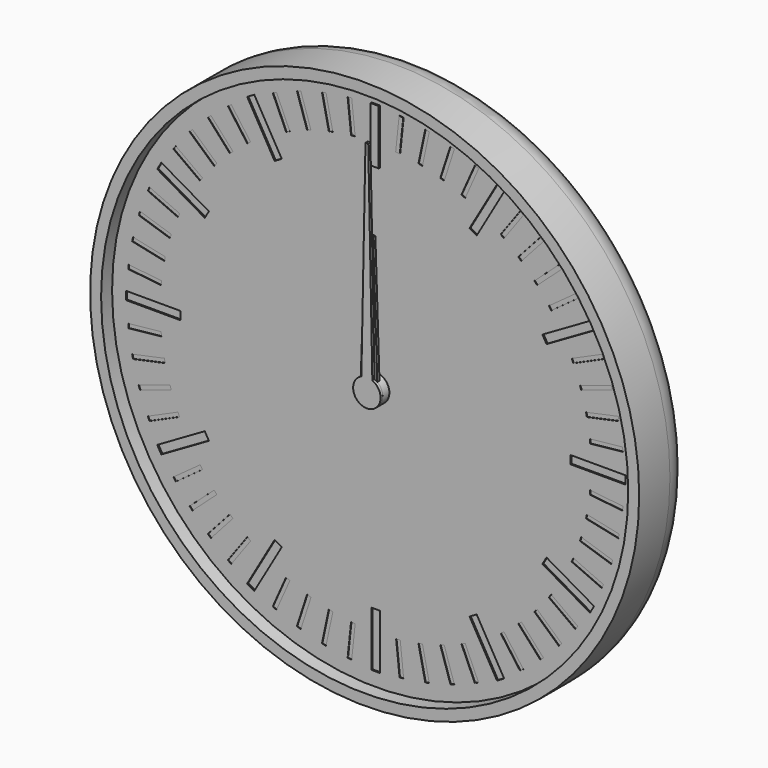
from build123d import *

# Parameters (mm, degrees)
F0_R      = 100
F1_DEPTH  = 24
F2_R      = 10
F3_T      = -4
F4_R      = 5
F4_R_2    = 3
F5_DEPTH  = 2
F6_DEPTH  = 19
F7_DEPTH  = 8
F9_DEPTH  = 4
F11_DEPTH = 4
F12_R     = 5
F12_R_2   = 3
F13_DEPTH = 2
F14_R     = 3
F15_DEPTH = 4
F17_DEPTH = 4
F18_R     = 3
F19_DEPTH = 2
F20_R     = 98
F20_R_2   = 5
F21_DEPTH = 1
F23_R     = 5
F23_R_2   = 3
F24_DEPTH = 2
F25_W     = 3
F25_H     = 20
F25_W_2   = 20
F25_H_2   = 3
F26_DEPTH = 0.5
F27_W     = 1.5
F27_H     = 12
F27_W_2   = 12
F27_H_2   = 1.5
F28_DEPTH = 0.2
F29_DEPTH = 1
F30_DEPTH = 0.4
F31_R     = 5
F31_R_2   = 3
F32_DEPTH = 5
F33_R     = 3
F34_DEPTH = 1
F36_DEPTH = 1


with BuildPart() as f1:
    # F0 (on Front) → F1 (new body)
    with BuildSketch(Plane.XZ):
        Circle(F0_R)
    extrude(amount=F1_DEPTH)

    # F2
    f2_edges = [f1.edges().sort_by_distance(p)[0] for p in [
        (-100, 0, 0),
    ]]
    fillet(f2_edges, radius=F2_R)

    # F3
    f3_openings = [f1.faces().sort_by_distance(p)[0] for p in [
        (0, -24, 0),
    ]]
    offset(amount=F3_T, openings=f3_openings)

    # F4 (on face) → F5 (join)
    with BuildSketch(Plane.XZ.offset(4)):
        Circle(F4_R)
        Circle(F4_R_2, mode=Mode.SUBTRACT)
        with Locations((40, 0)):
            Circle(F4_R)
        with Locations((40, 0)):
            Circle(F4_R_2, mode=Mode.SUBTRACT)
    extrude(amount=F5_DEPTH)


with BuildPart() as f6:
    # F6 (new): a face of the model
    f6_faces = [f1.part.faces().sort_by_distance(p)[0] for p in [
        (0, -4, 0),
    ]]
    extrude(f6_faces, amount=F6_DEPTH)

    # F8 (on face) → F9 (join)
    with BuildSketch(Plane.XZ.offset(6)):
        with BuildLine():
            ThreePointArc((9.2729637667, -1.3794085621), (9.3494561423, -0.6915886375), (9.375, 0))
            ThreePointArc((9.375, 0), (9.3494561423, 0.6915886375), (9.2729637667, 1.3794085621))
            ThreePointArc((9.2729637667, 1.3794085621), (8.9161548403, 2.8970343223), (8.3127812852, 4.3345463782))
            ThreePointArc((8.3127812852, 4.3345463782), (7.5845343223, 5.5104867402), (6.6911892658, 6.566476316))
            ThreePointArc((6.6911892658, 6.566476316), (5.5104867402, 7.5845343223), (4.1773988938, 8.3928519278))
            ThreePointArc((4.1773988938, 8.3928519278), (2.8970343223, 8.9161548403), (1.5536078905, 9.2453733036))
            ThreePointArc((1.5536078905, 9.2453733036), (0, 9.375), (-1.5536078905, 9.2453733036))
            ThreePointArc((-1.5536078905, 9.2453733036), (-2.8970343223, 8.9161548403), (-4.1773988938, 8.3928519278))
            ThreePointArc((-4.1773988938, 8.3928519278), (-5.5104867402, 7.5845343223), (-6.6911892658, 6.566476316))
            ThreePointArc((-6.6911892658, 6.566476316), (-7.5845343223, 5.5104867402), (-8.3127812852, 4.3345463782))
            ThreePointArc((-8.3127812852, 4.3345463782), (-8.9161548403, 2.8970343223), (-9.2729637667, 1.3794085621))
            ThreePointArc((-9.2729637667, 1.3794085621), (-9.375, 0), (-9.2729637667, -1.3794085621))
            ThreePointArc((-9.2729637667, -1.3794085621), (-8.9161548403, -2.8970343223), (-8.3127812852, -4.3345463782))
            ThreePointArc((-8.3127812852, -4.3345463782), (-7.5845343223, -5.5104867402), (-6.6911892658, -6.566476316))
            ThreePointArc((-6.6911892658, -6.566476316), (-5.5104867402, -7.5845343223), (-4.1773988938, -8.3928519278))
            ThreePointArc((-4.1773988938, -8.3928519278), (-2.8970343223, -8.9161548403), (-1.5536078905, -9.2453733036))
            ThreePointArc((-1.5536078905, -9.2453733036), (0, -9.375), (1.5536078905, -9.2453733036))
            ThreePointArc((1.5536078905, -9.2453733036), (2.8970343223, -8.9161548403), (4.1773988938, -8.3928519278))
            ThreePointArc((4.1773988938, -8.3928519278), (5.5104867402, -7.5845343223), (6.6911892658, -6.566476316))
            ThreePointArc((6.6911892658, -6.566476316), (7.5845343223, -5.5104867402), (8.3127812852, -4.3345463782))
            ThreePointArc((8.3127812852, -4.3345463782), (8.9161548403, -2.8970343223), (9.2729637667, -1.3794085621))
        make_face()
        with BuildLine():
            ThreePointArc((8.3127812852, 4.3345463782), (8.9161548403, 2.8970343223), (9.2729637667, 1.3794085621))
            Line((9.2729637667, 1.3794085621), (11.1823199426, 2.3946312492))
            Line((11.1823199426, 2.3946312492), (10.8182678729, 3.515068311))
            Line((10.8182678729, 3.515068311), (10.4542158031, 4.6355053728))
            Line((10.4542158031, 4.6355053728), (8.3127812852, 4.3345463782))
        make_face()
        with BuildLine():
            Line((11.1823199426, -2.3946312492), (9.2729637667, -1.3794085621))
            ThreePointArc((9.2729637667, -1.3794085621), (8.9161548403, -2.8970343223), (8.3127812852, -4.3345463782))
            Line((8.3127812852, -4.3345463782), (10.4542158031, -4.6355053728))
            Line((10.4542158031, -4.6355053728), (10.8182678729, -3.515068311))
            Line((10.8182678729, -3.515068311), (11.1823199426, -2.3946312492))
        make_face()
        with BuildLine():
            ThreePointArc((4.1773988938, 8.3928519278), (5.5104867402, 7.5845343223), (6.6911892658, 6.566476316))
            Line((6.6911892658, 6.566476316), (7.6391579371, 8.5101001246))
            Line((7.6391579371, 8.5101001246), (6.6860572448, 9.202568311))
            Line((6.6860572448, 9.202568311), (5.7329565525, 9.8950364974))
            Line((5.7329565525, 9.8950364974), (4.1773988938, 8.3928519278))
        make_face()
        with BuildLine():
            Line((7.6391579371, -8.5101001246), (6.6911892658, -6.566476316))
            ThreePointArc((6.6911892658, -6.566476316), (5.5104867402, -7.5845343223), (4.1773988938, -8.3928519278))
            Line((4.1773988938, -8.3928519278), (5.7329565525, -9.8950364974))
            Line((5.7329565525, -9.8950364974), (6.6860572448, -9.202568311))
            Line((6.6860572448, -9.202568311), (7.6391579371, -8.5101001246))
        make_face()
        with BuildLine():
            ThreePointArc((-1.5536078905, 9.2453733036), (0, 9.375), (1.5536078905, 9.2453733036))
            Line((1.5536078905, 9.2453733036), (1.1780972451, 11.375))
            Line((1.1780972451, 11.375), (0, 11.375))
            Line((0, 11.375), (-1.1780972451, 11.375))
            Line((-1.1780972451, 11.375), (-1.5536078905, 9.2453733036))
        make_face()
        with BuildLine():
            Line((1.1780972451, -11.375), (1.5536078905, -9.2453733036))
            ThreePointArc((1.5536078905, -9.2453733036), (0, -9.375), (-1.5536078905, -9.2453733036))
            Line((-1.5536078905, -9.2453733036), (-1.1780972451, -11.375))
            Line((-1.1780972451, -11.375), (0, -11.375))
            Line((0, -11.375), (1.1780972451, -11.375))
        make_face()
        with BuildLine():
            ThreePointArc((-6.6911892658, 6.566476316), (-5.5104867402, 7.5845343223), (-4.1773988938, 8.3928519278))
            Line((-4.1773988938, 8.3928519278), (-5.7329565525, 9.8950364974))
            Line((-5.7329565525, 9.8950364974), (-6.6860572448, 9.202568311))
            Line((-6.6860572448, 9.202568311), (-7.6391579371, 8.5101001246))
            Line((-7.6391579371, 8.5101001246), (-6.6911892658, 6.566476316))
        make_face()
        with BuildLine():
            Line((-5.7329565525, -9.8950364974), (-4.1773988938, -8.3928519278))
            ThreePointArc((-4.1773988938, -8.3928519278), (-5.5104867402, -7.5845343223), (-6.6911892658, -6.566476316))
            Line((-6.6911892658, -6.566476316), (-7.6391579371, -8.5101001246))
            Line((-7.6391579371, -8.5101001246), (-6.6860572448, -9.202568311))
            Line((-6.6860572448, -9.202568311), (-5.7329565525, -9.8950364974))
        make_face()
        with BuildLine():
            ThreePointArc((-9.2729637667, 1.3794085621), (-8.9161548403, 2.8970343223), (-8.3127812852, 4.3345463782))
            Line((-8.3127812852, 4.3345463782), (-10.4542158031, 4.6355053728))
            Line((-10.4542158031, 4.6355053728), (-10.8182678729, 3.515068311))
            Line((-10.8182678729, 3.515068311), (-11.1823199426, 2.3946312492))
            Line((-11.1823199426, 2.3946312492), (-9.2729637667, 1.3794085621))
        make_face()
        with BuildLine():
            Line((-10.4542158031, -4.6355053728), (-8.3127812852, -4.3345463782))
            ThreePointArc((-8.3127812852, -4.3345463782), (-8.9161548403, -2.8970343223), (-9.2729637667, -1.3794085621))
            Line((-9.2729637667, -1.3794085621), (-11.1823199426, -2.3946312492))
            Line((-11.1823199426, -2.3946312492), (-10.8182678729, -3.515068311))
            Line((-10.8182678729, -3.515068311), (-10.4542158031, -4.6355053728))
        make_face()
    extrude(amount=F9_DEPTH)

    # F35 (on face) → F36 (join)
    with BuildSketch(Plane.XZ.offset(23)):
        with BuildLine():
            ThreePointArc((-2, 4.582575695), (-2.7386127875, -4.1833001327), (5, 0))
            ThreePointArc((5, 0), (4.1833001327, 2.7386127875), (2, 4.582575695))
            ThreePointArc((2, 4.582575695), (0, 5), (-2, 4.582575695))
        make_face()
        with BuildLine():
            ThreePointArc((-2, 4.582575695), (0, 5), (2, 4.582575695))
            Line((2, 4.582575695), (0.5, 80))
            Line((0.5, 80), (0, 80))
            Line((0, 80), (-0.5, 80))
            Line((-0.5, 80), (-2, 4.582575695))
        make_face()
    extrude(amount=-F36_DEPTH)


with BuildPart() as f7:
    # F7 (new): a face of the model
    f7_faces = [f1.part.faces().sort_by_distance(p)[0] for p in [
        (40, -4, 0),
    ]]
    extrude(f7_faces, amount=F7_DEPTH)

    # F10 (on face) → F11 (join)
    with BuildSketch(Plane.XZ.offset(6)):
        with BuildLine():
            ThreePointArc((68.0829066802, -1.5381733945), (68.1144747006, -0.7693746225), (68.125, 0))
            ThreePointArc((68.125, 0), (68.1144747006, 0.7693746225), (68.0829066802, 1.5381733945))
            ThreePointArc((68.0829066802, 1.5381733945), (67.9709283072, 2.9398630294), (67.7890320221, 4.3342039956))
            ThreePointArc((67.7890320221, 4.3342039956), (67.5104012706, 5.8475163042), (67.1494235596, 7.3433252263))
            ThreePointArc((67.1494235596, 7.3433252263), (66.7484645208, 8.6911029668), (66.280643318, 10.0171558733))
            ThreePointArc((66.280643318, 10.0171558733), (65.6934659962, 11.4394680865), (65.0293803521, 12.8275385085))
            ThreePointArc((65.0293803521, 12.8275385085), (64.3569644814, 14.0625), (63.6236643925, 15.2623099717))
            ThreePointArc((63.6236643925, 15.2623099717), (62.7536029668, 16.5314602207), (61.815433119, 17.7511268046))
            ThreePointArc((61.815433119, 17.7511268046), (60.9009482166, 18.8192983038), (59.934217974, 19.8404278876))
            ThreePointArc((59.934217974, 19.8404278876), (58.8192983038, 20.9009482166), (57.6480467764, 21.8989056799))
            ThreePointArc((57.6480467764, 21.8989056799), (56.5314602207, 22.7536029668), (55.3735505752, 23.5514238999))
            ThreePointArc((55.3735505752, 23.5514238999), (54.0625, 24.3569644814), (52.709356105, 25.0895972944))
            ThreePointArc((52.709356105, 25.0895972944), (51.4394680865, 25.6934659962), (50.1409852457, 26.2331096755))
            ThreePointArc((50.1409852457, 26.2331096755), (48.6911029668, 26.7484645208), (47.2152055856, 27.1837531139))
            ThreePointArc((47.2152055856, 27.1837531139), (45.8475163042, 27.5104012706), (44.4652101991, 27.7682826779))
            ThreePointArc((44.4652101991, 27.7682826779), (42.9398630294, 27.9709283072), (41.4057159597, 28.0898484802))
            ThreePointArc((41.4057159597, 28.0898484802), (40, 28.125), (38.5942840403, 28.0898484802))
            ThreePointArc((38.5942840403, 28.0898484802), (37.0601369706, 27.9709283072), (35.5347898009, 27.7682826779))
            ThreePointArc((35.5347898009, 27.7682826779), (34.1524836958, 27.5104012706), (32.7847944144, 27.1837531139))
            ThreePointArc((32.7847944144, 27.1837531139), (31.3088970332, 26.7484645208), (29.8590147543, 26.2331096755))
            ThreePointArc((29.8590147543, 26.2331096755), (28.5605319135, 25.6934659962), (27.290643895, 25.0895972944))
            ThreePointArc((27.290643895, 25.0895972944), (25.9375, 24.3569644814), (24.6264494248, 23.5514238999))
            ThreePointArc((24.6264494248, 23.5514238999), (23.4685397793, 22.7536029668), (22.3519532236, 21.8989056799))
            ThreePointArc((22.3519532236, 21.8989056799), (21.1807016962, 20.9009482166), (20.065782026, 19.8404278876))
            ThreePointArc((20.065782026, 19.8404278876), (19.0990517834, 18.8192983038), (18.184566881, 17.7511268046))
            ThreePointArc((18.184566881, 17.7511268046), (17.2463970332, 16.5314602207), (16.3763356075, 15.2623099717))
            ThreePointArc((16.3763356075, 15.2623099717), (15.6430355186, 14.0625), (14.9706196479, 12.8275385085))
            ThreePointArc((14.9706196479, 12.8275385085), (14.3065340038, 11.4394680865), (13.719356682, 10.0171558733))
            ThreePointArc((13.719356682, 10.0171558733), (13.2515354792, 8.6911029668), (12.8505764404, 7.3433252263))
            ThreePointArc((12.8505764404, 7.3433252263), (12.4895987294, 5.8475163042), (12.2109679779, 4.3342039956))
            ThreePointArc((12.2109679779, 4.3342039956), (12.0290716928, 2.9398630294), (11.9170933198, 1.5381733945))
            ThreePointArc((11.9170933198, 1.5381733945), (11.875, 0), (11.9170933198, -1.5381733945))
            ThreePointArc((11.9170933198, -1.5381733945), (12.0290716928, -2.9398630294), (12.2109679779, -4.3342039956))
            ThreePointArc((12.2109679779, -4.3342039956), (12.4895987294, -5.8475163042), (12.8505764404, -7.3433252263))
            ThreePointArc((12.8505764404, -7.3433252263), (13.2515354792, -8.6911029668), (13.719356682, -10.0171558733))
            ThreePointArc((13.719356682, -10.0171558733), (14.3065340038, -11.4394680865), (14.9706196479, -12.8275385085))
            ThreePointArc((14.9706196479, -12.8275385085), (15.6430355186, -14.0625), (16.3763356075, -15.2623099717))
            ThreePointArc((16.3763356075, -15.2623099717), (17.2463970332, -16.5314602207), (18.184566881, -17.7511268046))
            ThreePointArc((18.184566881, -17.7511268046), (19.0990517834, -18.8192983038), (20.065782026, -19.8404278876))
            ThreePointArc((20.065782026, -19.8404278876), (21.1807016962, -20.9009482166), (22.3519532236, -21.8989056799))
            ThreePointArc((22.3519532236, -21.8989056799), (23.4685397793, -22.7536029668), (24.6264494248, -23.5514238999))
            ThreePointArc((24.6264494248, -23.5514238999), (25.9375, -24.3569644814), (27.290643895, -25.0895972944))
            ThreePointArc((27.290643895, -25.0895972944), (28.5605319135, -25.6934659962), (29.8590147543, -26.2331096755))
            ThreePointArc((29.8590147543, -26.2331096755), (31.3088970332, -26.7484645208), (32.7847944144, -27.1837531139))
            ThreePointArc((32.7847944144, -27.1837531139), (34.1524836958, -27.5104012706), (35.5347898009, -27.7682826779))
            ThreePointArc((35.5347898009, -27.7682826779), (37.0601369706, -27.9709283072), (38.5942840403, -28.0898484802))
            ThreePointArc((38.5942840403, -28.0898484802), (40, -28.125), (41.4057159597, -28.0898484802))
            ThreePointArc((41.4057159597, -28.0898484802), (42.9398630294, -27.9709283072), (44.4652101991, -27.7682826779))
            ThreePointArc((44.4652101991, -27.7682826779), (45.8475163042, -27.5104012706), (47.2152055856, -27.1837531139))
            ThreePointArc((47.2152055856, -27.1837531139), (48.6911029668, -26.7484645208), (50.1409852457, -26.2331096755))
            ThreePointArc((50.1409852457, -26.2331096755), (51.4394680865, -25.6934659962), (52.709356105, -25.0895972944))
            ThreePointArc((52.709356105, -25.0895972944), (54.0625, -24.3569644814), (55.3735505752, -23.5514238999))
            ThreePointArc((55.3735505752, -23.5514238999), (56.5314602207, -22.7536029668), (57.6480467764, -21.8989056799))
            ThreePointArc((57.6480467764, -21.8989056799), (58.8192983038, -20.9009482166), (59.934217974, -19.8404278876))
            ThreePointArc((59.934217974, -19.8404278876), (60.9009482166, -18.8192983038), (61.815433119, -17.7511268046))
            ThreePointArc((61.815433119, -17.7511268046), (62.7536029668, -16.5314602207), (63.6236643925, -15.2623099717))
            ThreePointArc((63.6236643925, -15.2623099717), (64.3569644814, -14.0625), (65.0293803521, -12.8275385085))
            ThreePointArc((65.0293803521, -12.8275385085), (65.6934659962, -11.4394680865), (66.280643318, -10.0171558733))
            ThreePointArc((66.280643318, -10.0171558733), (66.7484645208, -8.6911029668), (67.1494235596, -7.3433252263))
            ThreePointArc((67.1494235596, -7.3433252263), (67.5104012706, -5.8475163042), (67.7890320221, -4.3342039956))
            ThreePointArc((67.7890320221, -4.3342039956), (67.9709283072, -2.9398630294), (68.0829066802, -1.5381733945))
        make_face()
        with BuildLine():
            ThreePointArc((68.0829066802, 1.5381733945), (68.1144747006, 0.7693746225), (68.125, 0))
            ThreePointArc((68.125, 0), (68.1144747006, -0.7693746225), (68.0829066802, -1.5381733945))
            Line((68.0829066802, -1.5381733945), (70.125, -1.1780972451))
            Line((70.125, -1.1780972451), (70.125, 0))
            Line((70.125, 0), (70.125, 1.1780972451))
            Line((70.125, 1.1780972451), (68.0829066802, 1.5381733945))
        make_face()
        with BuildLine():
            ThreePointArc((67.1494235596, 7.3433252263), (67.5104012706, 5.8475163042), (67.7890320221, 4.3342039956))
            Line((67.7890320221, 4.3342039956), (69.7116366623, 5.1109866922))
            Line((69.7116366623, 5.1109866922), (69.4666964721, 6.2633396859))
            Line((69.4666964721, 6.2633396859), (69.2217562819, 7.4156926796))
            Line((69.2217562819, 7.4156926796), (67.1494235596, 7.3433252263))
        make_face()
        with BuildLine():
            Line((69.7116366623, -5.1109866922), (67.7890320221, -4.3342039956))
            ThreePointArc((67.7890320221, -4.3342039956), (67.5104012706, -5.8475163042), (67.1494235596, -7.3433252263))
            Line((67.1494235596, -7.3433252263), (69.2217562819, -7.4156926796))
            Line((69.2217562819, -7.4156926796), (69.4666964721, -6.2633396859))
            Line((69.4666964721, -6.2633396859), (69.7116366623, -5.1109866922))
        make_face()
        with BuildLine():
            ThreePointArc((65.0293803521, 12.8275385085), (65.6934659962, 11.4394680865), (66.280643318, 10.0171558733))
            Line((66.280643318, 10.0171558733), (67.9997322302, 11.1766959857))
            Line((67.9997322302, 11.1766959857), (67.5205569115, 12.2529413727))
            Line((67.5205569115, 12.2529413727), (67.0413815928, 13.3291867596))
            Line((67.0413815928, 13.3291867596), (65.0293803521, 12.8275385085))
        make_face()
        with BuildLine():
            Line((67.9997322302, -11.1766959857), (66.280643318, -10.0171558733))
            ThreePointArc((66.280643318, -10.0171558733), (65.6934659962, -11.4394680865), (65.0293803521, -12.8275385085))
            Line((65.0293803521, -12.8275385085), (67.0413815928, -13.3291867596))
            Line((67.0413815928, -13.3291867596), (67.5205569115, -12.2529413727))
            Line((67.5205569115, -12.2529413727), (67.9997322302, -11.1766959857))
        make_face()
        with BuildLine():
            ThreePointArc((61.815433119, 17.7511268046), (62.7536029668, 16.5314602207), (63.6236643925, 15.2623099717))
            Line((63.6236643925, 15.2623099717), (65.064105142, 16.753930033))
            Line((65.064105142, 16.753930033), (64.3716369555, 17.7070307253))
            Line((64.3716369555, 17.7070307253), (63.6791687691, 18.6601314176))
            Line((63.6791687691, 18.6601314176), (61.815433119, 17.7511268046))
        make_face()
        with BuildLine():
            Line((65.064105142, -16.753930033), (63.6236643925, -15.2623099717))
            ThreePointArc((63.6236643925, -15.2623099717), (62.7536029668, -16.5314602207), (61.815433119, -17.7511268046))
            Line((61.815433119, -17.7511268046), (63.6791687691, -18.6601314176))
            Line((63.6791687691, -18.6601314176), (64.3716369555, -17.7070307253))
            Line((64.3716369555, -17.7070307253), (65.064105142, -16.753930033))
        make_face()
        with BuildLine():
            ThreePointArc((57.6480467764, 21.8989056799), (58.8192983038, 20.9009482166), (59.934217974, 19.8404278876))
            Line((59.934217974, 19.8404278876), (61.0330563882, 21.5989369435))
            Line((61.0330563882, 21.5989369435), (60.1575595166, 22.3872378675))
            Line((60.1575595166, 22.3872378675), (59.282062645, 23.1755387915))
            Line((59.282062645, 23.1755387915), (57.6480467764, 21.8989056799))
        make_face()
        with BuildLine():
            Line((61.0330563882, -21.5989369435), (59.934217974, -19.8404278876))
            ThreePointArc((59.934217974, -19.8404278876), (58.8192983038, -20.9009482166), (57.6480467764, -21.8989056799))
            Line((57.6480467764, -21.8989056799), (59.282062645, -23.1755387915))
            Line((59.282062645, -23.1755387915), (60.1575595166, -22.3872378675))
            Line((60.1575595166, -22.3872378675), (61.0330563882, -21.5989369435))
        make_face()
        with BuildLine():
            ThreePointArc((52.709356105, 25.0895972944), (54.0625, 24.3569644814), (55.3735505752, 23.5514238999))
            Line((55.3735505752, 23.5514238999), (56.0827621424, 25.4999666665))
            Line((56.0827621424, 25.4999666665), (55.0625, 26.089015289))
            Line((55.0625, 26.089015289), (54.0422378576, 26.6780639116))
            Line((54.0422378576, 26.6780639116), (52.709356105, 25.0895972944))
        make_face()
        with BuildLine():
            Line((56.0827621424, -25.4999666665), (55.3735505752, -23.5514238999))
            ThreePointArc((55.3735505752, -23.5514238999), (54.0625, -24.3569644814), (52.709356105, -25.0895972944))
            Line((52.709356105, -25.0895972944), (54.0422378576, -26.6780639116))
            Line((54.0422378576, -26.6780639116), (55.0625, -26.089015289))
            Line((55.0625, -26.089015289), (56.0827621424, -25.4999666665))
        make_face()
        with BuildLine():
            ThreePointArc((47.2152055856, 27.1837531139), (48.6911029668, 26.7484645208), (50.1409852457, 26.2331096755))
            Line((50.1409852457, 26.2331096755), (50.4295740173, 28.2865254836))
            Line((50.4295740173, 28.2865254836), (49.3091369555, 28.6505775534))
            Line((49.3091369555, 28.6505775534), (48.1886998938, 29.0146296232))
            Line((48.1886998938, 29.0146296232), (47.2152055856, 27.1837531139))
        make_face()
        with BuildLine():
            Line((50.4295740173, -28.2865254836), (50.1409852457, -26.2331096755))
            ThreePointArc((50.1409852457, -26.2331096755), (48.6911029668, -26.7484645208), (47.2152055856, -27.1837531139))
            Line((47.2152055856, -27.1837531139), (48.1886998938, -29.0146296232))
            Line((48.1886998938, -29.0146296232), (49.3091369555, -28.6505775534))
            Line((49.3091369555, -28.6505775534), (50.4295740173, -28.2865254836))
        make_face()
        with BuildLine():
            ThreePointArc((41.4057159597, 28.0898484802), (42.9398630294, 27.9709283072), (44.4652101991, 27.7682826779))
            Line((44.4652101991, 27.7682826779), (44.3205634611, 29.8368274034))
            Line((44.3205634611, 29.8368274034), (43.1489199559, 29.959972098))
            Line((43.1489199559, 29.959972098), (41.9772764508, 30.0831167926))
            Line((41.9772764508, 30.0831167926), (41.4057159597, 28.0898484802))
        make_face()
        with BuildLine():
            Line((44.3205634611, -29.8368274034), (44.4652101991, -27.7682826779))
            ThreePointArc((44.4652101991, -27.7682826779), (42.9398630294, -27.9709283072), (41.4057159597, -28.0898484802))
            Line((41.4057159597, -28.0898484802), (41.9772764508, -30.0831167926))
            Line((41.9772764508, -30.0831167926), (43.1489199559, -29.959972098))
            Line((43.1489199559, -29.959972098), (44.3205634611, -29.8368274034))
        make_face()
        with BuildLine():
            ThreePointArc((35.5347898009, 27.7682826779), (37.0601369706, 27.9709283072), (38.5942840403, 28.0898484802))
            Line((38.5942840403, 28.0898484802), (38.0227235492, 30.0831167926))
            Line((38.0227235492, 30.0831167926), (36.8510800441, 29.959972098))
            Line((36.8510800441, 29.959972098), (35.6794365389, 29.8368274034))
            Line((35.6794365389, 29.8368274034), (35.5347898009, 27.7682826779))
        make_face()
        with BuildLine():
            Line((38.0227235492, -30.0831167926), (38.5942840403, -28.0898484802))
            ThreePointArc((38.5942840403, -28.0898484802), (37.0601369706, -27.9709283072), (35.5347898009, -27.7682826779))
            Line((35.5347898009, -27.7682826779), (35.6794365389, -29.8368274034))
            Line((35.6794365389, -29.8368274034), (36.8510800441, -29.959972098))
            Line((36.8510800441, -29.959972098), (38.0227235492, -30.0831167926))
        make_face()
        with BuildLine():
            ThreePointArc((29.8590147543, 26.2331096755), (31.3088970332, 26.7484645208), (32.7847944144, 27.1837531139))
            Line((32.7847944144, 27.1837531139), (31.8113001062, 29.0146296232))
            Line((31.8113001062, 29.0146296232), (30.6908630445, 28.6505775534))
            Line((30.6908630445, 28.6505775534), (29.5704259827, 28.2865254836))
            Line((29.5704259827, 28.2865254836), (29.8590147543, 26.2331096755))
        make_face()
        with BuildLine():
            Line((31.8113001062, -29.0146296232), (32.7847944144, -27.1837531139))
            ThreePointArc((32.7847944144, -27.1837531139), (31.3088970332, -26.7484645208), (29.8590147543, -26.2331096755))
            Line((29.8590147543, -26.2331096755), (29.5704259827, -28.2865254836))
            Line((29.5704259827, -28.2865254836), (30.6908630445, -28.6505775534))
            Line((30.6908630445, -28.6505775534), (31.8113001062, -29.0146296232))
        make_face()
        with BuildLine():
            ThreePointArc((24.6264494248, 23.5514238999), (25.9375, 24.3569644814), (27.290643895, 25.0895972944))
            Line((27.290643895, 25.0895972944), (25.9577621424, 26.6780639116))
            Line((25.9577621424, 26.6780639116), (24.9375, 26.089015289))
            Line((24.9375, 26.089015289), (23.9172378576, 25.4999666665))
            Line((23.9172378576, 25.4999666665), (24.6264494248, 23.5514238999))
        make_face()
        with BuildLine():
            Line((25.9577621424, -26.6780639116), (27.290643895, -25.0895972944))
            ThreePointArc((27.290643895, -25.0895972944), (25.9375, -24.3569644814), (24.6264494248, -23.5514238999))
            Line((24.6264494248, -23.5514238999), (23.9172378576, -25.4999666665))
            Line((23.9172378576, -25.4999666665), (24.9375, -26.089015289))
            Line((24.9375, -26.089015289), (25.9577621424, -26.6780639116))
        make_face()
        with BuildLine():
            ThreePointArc((20.065782026, 19.8404278876), (21.1807016962, 20.9009482166), (22.3519532236, 21.8989056799))
            Line((22.3519532236, 21.8989056799), (20.717937355, 23.1755387915))
            Line((20.717937355, 23.1755387915), (19.8424404834, 22.3872378675))
            Line((19.8424404834, 22.3872378675), (18.9669436118, 21.5989369435))
            Line((18.9669436118, 21.5989369435), (20.065782026, 19.8404278876))
        make_face()
        with BuildLine():
            Line((20.717937355, -23.1755387915), (22.3519532236, -21.8989056799))
            ThreePointArc((22.3519532236, -21.8989056799), (21.1807016962, -20.9009482166), (20.065782026, -19.8404278876))
            Line((20.065782026, -19.8404278876), (18.9669436118, -21.5989369435))
            Line((18.9669436118, -21.5989369435), (19.8424404834, -22.3872378675))
            Line((19.8424404834, -22.3872378675), (20.717937355, -23.1755387915))
        make_face()
        with BuildLine():
            ThreePointArc((16.3763356075, 15.2623099717), (17.2463970332, 16.5314602207), (18.184566881, 17.7511268046))
            Line((18.184566881, 17.7511268046), (16.3208312309, 18.6601314176))
            Line((16.3208312309, 18.6601314176), (15.6283630445, 17.7070307253))
            Line((15.6283630445, 17.7070307253), (14.935894858, 16.753930033))
            Line((14.935894858, 16.753930033), (16.3763356075, 15.2623099717))
        make_face()
        with BuildLine():
            Line((16.3208312309, -18.6601314176), (18.184566881, -17.7511268046))
            ThreePointArc((18.184566881, -17.7511268046), (17.2463970332, -16.5314602207), (16.3763356075, -15.2623099717))
            Line((16.3763356075, -15.2623099717), (14.935894858, -16.753930033))
            Line((14.935894858, -16.753930033), (15.6283630445, -17.7070307253))
            Line((15.6283630445, -17.7070307253), (16.3208312309, -18.6601314176))
        make_face()
        with BuildLine():
            ThreePointArc((13.719356682, 10.0171558733), (14.3065340038, 11.4394680865), (14.9706196479, 12.8275385085))
            Line((14.9706196479, 12.8275385085), (12.9586184072, 13.3291867596))
            Line((12.9586184072, 13.3291867596), (12.4794430885, 12.2529413727))
            Line((12.4794430885, 12.2529413727), (12.0002677698, 11.1766959857))
            Line((12.0002677698, 11.1766959857), (13.719356682, 10.0171558733))
        make_face()
        with BuildLine():
            Line((12.9586184072, -13.3291867596), (14.9706196479, -12.8275385085))
            ThreePointArc((14.9706196479, -12.8275385085), (14.3065340038, -11.4394680865), (13.719356682, -10.0171558733))
            Line((13.719356682, -10.0171558733), (12.0002677698, -11.1766959857))
            Line((12.0002677698, -11.1766959857), (12.4794430885, -12.2529413727))
            Line((12.4794430885, -12.2529413727), (12.9586184072, -13.3291867596))
        make_face()
        with BuildLine():
            ThreePointArc((12.2109679779, 4.3342039956), (12.4895987294, 5.8475163042), (12.8505764404, 7.3433252263))
            Line((12.8505764404, 7.3433252263), (10.7782437181, 7.4156926796))
            Line((10.7782437181, 7.4156926796), (10.5333035279, 6.2633396859))
            Line((10.5333035279, 6.2633396859), (10.2883633377, 5.1109866922))
            Line((10.2883633377, 5.1109866922), (12.2109679779, 4.3342039956))
        make_face()
        with BuildLine():
            Line((10.7782437181, -7.4156926796), (12.8505764404, -7.3433252263))
            ThreePointArc((12.8505764404, -7.3433252263), (12.4895987294, -5.8475163042), (12.2109679779, -4.3342039956))
            Line((12.2109679779, -4.3342039956), (10.2883633377, -5.1109866922))
            Line((10.2883633377, -5.1109866922), (10.5333035279, -6.2633396859))
            Line((10.5333035279, -6.2633396859), (10.7782437181, -7.4156926796))
        make_face()
        with BuildLine():
            ThreePointArc((11.9170933198, -1.5381733945), (11.875, 0), (11.9170933198, 1.5381733945))
            Line((11.9170933198, 1.5381733945), (9.875, 1.1780972451))
            Line((9.875, 1.1780972451), (9.875, 0))
            Line((9.875, 0), (9.875, -1.1780972451))
            Line((9.875, -1.1780972451), (11.9170933198, -1.5381733945))
        make_face()
    extrude(amount=F11_DEPTH)

    # F16 (on face) → F17 (join)
    with BuildSketch(Plane.XZ.offset(12)):
        with BuildLine():
            ThreePointArc((47.4288750323, -1.0304444454), (47.4821976298, -0.5164480894), (47.5, 0))
            ThreePointArc((47.5, 0), (47.4821976298, 0.5164480894), (47.4288750323, 1.0304444454))
            ThreePointArc((47.4288750323, 1.0304444454), (47.1329238722, 2.3176274578), (46.6157661985, 3.532936117))
            ThreePointArc((46.6157661985, 3.532936117), (46.0676274578, 4.4083893922), (45.4044061018, 5.2002302532))
            ThreePointArc((45.4044061018, 5.2002302532), (44.4083893922, 6.0676274578), (43.2756595386, 6.7468551628))
            ThreePointArc((43.2756595386, 6.7468551628), (42.3176274578, 7.1329238722), (41.3156377295, 7.3837048536))
            ThreePointArc((41.3156377295, 7.3837048536), (40, 7.5), (38.6843622705, 7.3837048536))
            ThreePointArc((38.6843622705, 7.3837048536), (37.6823725422, 7.1329238722), (36.7243404614, 6.7468551628))
            ThreePointArc((36.7243404614, 6.7468551628), (35.5916106078, 6.0676274578), (34.5955938982, 5.2002302532))
            ThreePointArc((34.5955938982, 5.2002302532), (33.9323725422, 4.4083893922), (33.3842338015, 3.532936117))
            ThreePointArc((33.3842338015, 3.532936117), (32.8670761278, 2.3176274578), (32.5711249677, 1.0304444454))
            ThreePointArc((32.5711249677, 1.0304444454), (32.5, 0), (32.5711249677, -1.0304444454))
            ThreePointArc((32.5711249677, -1.0304444454), (32.8670761278, -2.3176274578), (33.3842338015, -3.532936117))
            ThreePointArc((33.3842338015, -3.532936117), (33.9323725422, -4.4083893922), (34.5955938982, -5.2002302532))
            ThreePointArc((34.5955938982, -5.2002302532), (35.5916106078, -6.0676274578), (36.7243404614, -6.7468551628))
            ThreePointArc((36.7243404614, -6.7468551628), (37.6823725422, -7.1329238722), (38.6843622705, -7.3837048536))
            ThreePointArc((38.6843622705, -7.3837048536), (40, -7.5), (41.3156377295, -7.3837048536))
            ThreePointArc((41.3156377295, -7.3837048536), (42.3176274578, -7.1329238722), (43.2756595386, -6.7468551628))
            ThreePointArc((43.2756595386, -6.7468551628), (44.4083893922, -6.0676274578), (45.4044061018, -5.2002302532))
            ThreePointArc((45.4044061018, -5.2002302532), (46.0676274578, -4.4083893922), (46.6157661985, -3.532936117))
            ThreePointArc((46.6157661985, -3.532936117), (47.1329238722, -2.3176274578), (47.4288750323, -1.0304444454))
        make_face()
        with BuildLine():
            ThreePointArc((46.6157661985, 3.532936117), (47.1329238722, 2.3176274578), (47.4288750323, 1.0304444454))
            Line((47.4288750323, 1.0304444454), (49.3262785606, 2.0393117971))
            Line((49.3262785606, 2.0393117971), (48.743795249, 3.832011096))
            Line((48.743795249, 3.832011096), (46.6157661985, 3.532936117))
        make_face()
        with BuildLine():
            Line((49.3262785606, -2.0393117971), (47.4288750323, -1.0304444454))
            ThreePointArc((47.4288750323, -1.0304444454), (47.1329238722, -2.3176274578), (46.6157661985, -3.532936117))
            Line((46.6157661985, -3.532936117), (48.743795249, -3.832011096))
            Line((48.743795249, -3.832011096), (49.3262785606, -2.0393117971))
        make_face()
        with BuildLine():
            ThreePointArc((43.2756595386, 6.7468551628), (44.4083893922, 6.0676274578), (45.4044061018, 5.2002302532))
            Line((45.4044061018, 5.2002302532), (46.3464404506, 7.1316868974))
            Line((46.3464404506, 7.1316868974), (44.8214793429, 8.2396359957))
            Line((44.8214793429, 8.2396359957), (43.2756595386, 6.7468551628))
        make_face()
        with BuildLine():
            Line((46.3464404506, -7.1316868974), (45.4044061018, -5.2002302532))
            ThreePointArc((45.4044061018, -5.2002302532), (44.4083893922, -6.0676274578), (43.2756595386, -6.7468551628))
            Line((43.2756595386, -6.7468551628), (44.8214793429, -8.2396359957))
            Line((44.8214793429, -8.2396359957), (46.3464404506, -7.1316868974))
        make_face()
        with BuildLine():
            ThreePointArc((38.6843622705, 7.3837048536), (40, 7.5), (41.3156377295, 7.3837048536))
            Line((41.3156377295, 7.3837048536), (40.9424777961, 9.5))
            Line((40.9424777961, 9.5), (39.0575222039, 9.5))
            Line((39.0575222039, 9.5), (38.6843622705, 7.3837048536))
        make_face()
        with BuildLine():
            Line((40.9424777961, -9.5), (41.3156377295, -7.3837048536))
            ThreePointArc((41.3156377295, -7.3837048536), (40, -7.5), (38.6843622705, -7.3837048536))
            Line((38.6843622705, -7.3837048536), (39.0575222039, -9.5))
            Line((39.0575222039, -9.5), (40.9424777961, -9.5))
        make_face()
        with BuildLine():
            ThreePointArc((34.5955938982, 5.2002302532), (35.5916106078, 6.0676274578), (36.7243404614, 6.7468551628))
            Line((36.7243404614, 6.7468551628), (35.1785206571, 8.2396359957))
            Line((35.1785206571, 8.2396359957), (33.6535595494, 7.1316868974))
            Line((33.6535595494, 7.1316868974), (34.5955938982, 5.2002302532))
        make_face()
        with BuildLine():
            Line((35.1785206571, -8.2396359957), (36.7243404614, -6.7468551628))
            ThreePointArc((36.7243404614, -6.7468551628), (35.5916106078, -6.0676274578), (34.5955938982, -5.2002302532))
            Line((34.5955938982, -5.2002302532), (33.6535595494, -7.1316868974))
            Line((33.6535595494, -7.1316868974), (35.1785206571, -8.2396359957))
        make_face()
        with BuildLine():
            ThreePointArc((32.5711249677, 1.0304444454), (32.8670761278, 2.3176274578), (33.3842338015, 3.532936117))
            Line((33.3842338015, 3.532936117), (31.256204751, 3.832011096))
            Line((31.256204751, 3.832011096), (30.6737214394, 2.0393117971))
            Line((30.6737214394, 2.0393117971), (32.5711249677, 1.0304444454))
        make_face()
        with BuildLine():
            Line((31.256204751, -3.832011096), (33.3842338015, -3.532936117))
            ThreePointArc((33.3842338015, -3.532936117), (32.8670761278, -2.3176274578), (32.5711249677, -1.0304444454))
            Line((32.5711249677, -1.0304444454), (30.6737214394, -2.0393117971))
            Line((30.6737214394, -2.0393117971), (31.256204751, -3.832011096))
        make_face()
    extrude(amount=F17_DEPTH)

    # F18 (on face) → F19 (join)
    with BuildSketch(Plane.XZ.offset(16)):
        with Locations((40, 0)):
            Circle(F18_R)
    extrude(amount=F19_DEPTH)


with BuildPart() as f13:
    # F12 (on face) → F13 (new body)
    with BuildSketch(Plane.XZ.offset(10)):
        Circle(F12_R)
        Circle(F12_R_2, mode=Mode.SUBTRACT)
    extrude(amount=F13_DEPTH)

    # F14 (on face) → F15 (join)
    with BuildSketch(Plane.XZ.offset(12)):
        with BuildLine():
            ThreePointArc((29.9718156995, -1.3001014101), (29.9929530972, -0.6502034357), (30, 0))
            ThreePointArc((30, 0), (29.9929530972, 0.6502034357), (29.9718156995, 1.3001014101))
            ThreePointArc((29.9718156995, 1.3001014101), (29.907520012, 2.3537728718), (29.8061935814, 3.4045299509))
            ThreePointArc((29.8061935814, 3.4045299509), (29.6306502179, 4.6930339512), (29.3994322443, 5.9727199596))
            ThreePointArc((29.3994322443, 5.9727199596), (29.1710976119, 7.0033609157), (28.9066440563, 8.0253304855))
            ThreePointArc((28.9066440563, 8.0253304855), (28.5316954889, 9.2705098312), (28.1031371961, 10.4982703213))
            ThreePointArc((28.1031371961, 10.4982703213), (27.7163859753, 11.480502971), (27.2953170189, 12.448520749))
            ThreePointArc((27.2953170189, 12.448520749), (26.7301957257, 13.6197149922), (26.1148496411, 14.765318426))
            ThreePointArc((26.1148496411, 14.765318426), (25.5792049306, 15.6749569415), (25.0118886885, 16.5651871174))
            ThreePointArc((25.0118886885, 16.5651871174), (24.2705098312, 17.6335575688), (23.4835278178, 18.6687953878))
            ThreePointArc((23.4835278178, 18.6687953878), (22.812178968, 19.4834414499), (22.1125846489, 20.2739636023))
            ThreePointArc((22.1125846489, 20.2739636023), (21.2132034356, 21.2132034356), (20.2739636023, 22.1125846489))
            ThreePointArc((20.2739636023, 22.1125846489), (19.4834414499, 22.812178968), (18.6687953878, 23.4835278178))
            ThreePointArc((18.6687953878, 23.4835278178), (17.6335575688, 24.2705098312), (16.5651871174, 25.0118886885))
            ThreePointArc((16.5651871174, 25.0118886885), (15.6749569415, 25.5792049306), (14.765318426, 26.1148496411))
            ThreePointArc((14.765318426, 26.1148496411), (13.6197149922, 26.7301957257), (12.448520749, 27.2953170189))
            ThreePointArc((12.448520749, 27.2953170189), (11.480502971, 27.7163859753), (10.4982703213, 28.1031371961))
            ThreePointArc((10.4982703213, 28.1031371961), (9.2705098312, 28.5316954889), (8.0253304855, 28.9066440563))
            ThreePointArc((8.0253304855, 28.9066440563), (7.0033609157, 29.1710976119), (5.9727199596, 29.3994322443))
            ThreePointArc((5.9727199596, 29.3994322443), (4.6930339512, 29.6306502179), (3.4045299509, 29.8061935814))
            ThreePointArc((3.4045299509, 29.8061935814), (2.3537728718, 29.907520012), (1.3001014101, 29.9718156995))
            ThreePointArc((1.3001014101, 29.9718156995), (0, 30), (-1.3001014101, 29.9718156995))
            ThreePointArc((-1.3001014101, 29.9718156995), (-2.3537728718, 29.907520012), (-3.4045299509, 29.8061935814))
            ThreePointArc((-3.4045299509, 29.8061935814), (-4.6930339512, 29.6306502179), (-5.9727199596, 29.3994322443))
            ThreePointArc((-5.9727199596, 29.3994322443), (-7.0033609157, 29.1710976119), (-8.0253304855, 28.9066440563))
            ThreePointArc((-8.0253304855, 28.9066440563), (-9.2705098312, 28.5316954889), (-10.4982703213, 28.1031371961))
            ThreePointArc((-10.4982703213, 28.1031371961), (-11.480502971, 27.7163859753), (-12.448520749, 27.2953170189))
            ThreePointArc((-12.448520749, 27.2953170189), (-13.6197149922, 26.7301957257), (-14.765318426, 26.1148496411))
            ThreePointArc((-14.765318426, 26.1148496411), (-15.6749569415, 25.5792049306), (-16.5651871174, 25.0118886885))
            ThreePointArc((-16.5651871174, 25.0118886885), (-17.6335575688, 24.2705098312), (-18.6687953878, 23.4835278178))
            ThreePointArc((-18.6687953878, 23.4835278178), (-19.4834414499, 22.812178968), (-20.2739636023, 22.1125846489))
            ThreePointArc((-20.2739636023, 22.1125846489), (-21.2132034356, 21.2132034356), (-22.1125846489, 20.2739636023))
            ThreePointArc((-22.1125846489, 20.2739636023), (-22.812178968, 19.4834414499), (-23.4835278178, 18.6687953878))
            ThreePointArc((-23.4835278178, 18.6687953878), (-24.2705098312, 17.6335575688), (-25.0118886885, 16.5651871174))
            ThreePointArc((-25.0118886885, 16.5651871174), (-25.5792049306, 15.6749569415), (-26.1148496411, 14.765318426))
            ThreePointArc((-26.1148496411, 14.765318426), (-26.7301957257, 13.6197149922), (-27.2953170189, 12.448520749))
            ThreePointArc((-27.2953170189, 12.448520749), (-27.7163859753, 11.480502971), (-28.1031371961, 10.4982703213))
            ThreePointArc((-28.1031371961, 10.4982703213), (-28.5316954889, 9.2705098312), (-28.9066440563, 8.0253304855))
            ThreePointArc((-28.9066440563, 8.0253304855), (-29.1710976119, 7.0033609157), (-29.3994322443, 5.9727199596))
            ThreePointArc((-29.3994322443, 5.9727199596), (-29.6306502179, 4.6930339512), (-29.8061935814, 3.4045299509))
            ThreePointArc((-29.8061935814, 3.4045299509), (-29.907520012, 2.3537728718), (-29.9718156995, 1.3001014101))
            ThreePointArc((-29.9718156995, 1.3001014101), (-30, 0), (-29.9718156995, -1.3001014101))
            ThreePointArc((-29.9718156995, -1.3001014101), (-29.907520012, -2.3537728718), (-29.8061935814, -3.4045299509))
            ThreePointArc((-29.8061935814, -3.4045299509), (-29.6306502179, -4.6930339512), (-29.3994322443, -5.9727199596))
            ThreePointArc((-29.3994322443, -5.9727199596), (-29.1710976119, -7.0033609157), (-28.9066440563, -8.0253304855))
            ThreePointArc((-28.9066440563, -8.0253304855), (-28.5316954889, -9.2705098312), (-28.1031371961, -10.4982703213))
            ThreePointArc((-28.1031371961, -10.4982703213), (-27.7163859753, -11.480502971), (-27.2953170189, -12.448520749))
            ThreePointArc((-27.2953170189, -12.448520749), (-26.7301957257, -13.6197149922), (-26.1148496411, -14.765318426))
            ThreePointArc((-26.1148496411, -14.765318426), (-25.5792049306, -15.6749569415), (-25.0118886885, -16.5651871174))
            ThreePointArc((-25.0118886885, -16.5651871174), (-24.2705098312, -17.6335575688), (-23.4835278178, -18.6687953878))
            ThreePointArc((-23.4835278178, -18.6687953878), (-22.812178968, -19.4834414499), (-22.1125846489, -20.2739636023))
            ThreePointArc((-22.1125846489, -20.2739636023), (-21.2132034356, -21.2132034356), (-20.2739636023, -22.1125846489))
            ThreePointArc((-20.2739636023, -22.1125846489), (-19.4834414499, -22.812178968), (-18.6687953878, -23.4835278178))
            ThreePointArc((-18.6687953878, -23.4835278178), (-17.6335575688, -24.2705098312), (-16.5651871174, -25.0118886885))
            ThreePointArc((-16.5651871174, -25.0118886885), (-15.6749569415, -25.5792049306), (-14.765318426, -26.1148496411))
            ThreePointArc((-14.765318426, -26.1148496411), (-13.6197149922, -26.7301957257), (-12.448520749, -27.2953170189))
            ThreePointArc((-12.448520749, -27.2953170189), (-11.480502971, -27.7163859753), (-10.4982703213, -28.1031371961))
            ThreePointArc((-10.4982703213, -28.1031371961), (-9.2705098312, -28.5316954889), (-8.0253304855, -28.9066440563))
            ThreePointArc((-8.0253304855, -28.9066440563), (-7.0033609157, -29.1710976119), (-5.9727199596, -29.3994322443))
            ThreePointArc((-5.9727199596, -29.3994322443), (-4.6930339512, -29.6306502179), (-3.4045299509, -29.8061935814))
            ThreePointArc((-3.4045299509, -29.8061935814), (-2.3537728718, -29.907520012), (-1.3001014101, -29.9718156995))
            ThreePointArc((-1.3001014101, -29.9718156995), (0, -30), (1.3001014101, -29.9718156995))
            ThreePointArc((1.3001014101, -29.9718156995), (2.3537728718, -29.907520012), (3.4045299509, -29.8061935814))
            ThreePointArc((3.4045299509, -29.8061935814), (4.6930339512, -29.6306502179), (5.9727199596, -29.3994322443))
            ThreePointArc((5.9727199596, -29.3994322443), (7.0033609157, -29.1710976119), (8.0253304855, -28.9066440563))
            ThreePointArc((8.0253304855, -28.9066440563), (9.2705098312, -28.5316954889), (10.4982703213, -28.1031371961))
            ThreePointArc((10.4982703213, -28.1031371961), (11.480502971, -27.7163859753), (12.448520749, -27.2953170189))
            ThreePointArc((12.448520749, -27.2953170189), (13.6197149922, -26.7301957257), (14.765318426, -26.1148496411))
            ThreePointArc((14.765318426, -26.1148496411), (15.6749569415, -25.5792049306), (16.5651871174, -25.0118886885))
            ThreePointArc((16.5651871174, -25.0118886885), (17.6335575688, -24.2705098312), (18.6687953878, -23.4835278178))
            ThreePointArc((18.6687953878, -23.4835278178), (19.4834414499, -22.812178968), (20.2739636023, -22.1125846489))
            ThreePointArc((20.2739636023, -22.1125846489), (21.2132034356, -21.2132034356), (22.1125846489, -20.2739636023))
            ThreePointArc((22.1125846489, -20.2739636023), (22.812178968, -19.4834414499), (23.4835278178, -18.6687953878))
            ThreePointArc((23.4835278178, -18.6687953878), (24.2705098312, -17.6335575688), (25.0118886885, -16.5651871174))
            ThreePointArc((25.0118886885, -16.5651871174), (25.5792049306, -15.6749569415), (26.1148496411, -14.765318426))
            ThreePointArc((26.1148496411, -14.765318426), (26.7301957257, -13.6197149922), (27.2953170189, -12.448520749))
            ThreePointArc((27.2953170189, -12.448520749), (27.7163859753, -11.480502971), (28.1031371961, -10.4982703213))
            ThreePointArc((28.1031371961, -10.4982703213), (28.5316954889, -9.2705098312), (28.9066440563, -8.0253304855))
            ThreePointArc((28.9066440563, -8.0253304855), (29.1710976119, -7.0033609157), (29.3994322443, -5.9727199596))
            ThreePointArc((29.3994322443, -5.9727199596), (29.6306502179, -4.6930339512), (29.8061935814, -3.4045299509))
            ThreePointArc((29.8061935814, -3.4045299509), (29.907520012, -2.3537728718), (29.9718156995, -1.3001014101))
        make_face()
        Circle(F14_R, mode=Mode.SUBTRACT)
        with BuildLine():
            ThreePointArc((29.9718156995, 1.3001014101), (29.9929530972, 0.6502034357), (30, 0))
            ThreePointArc((30, 0), (29.9929530972, -0.6502034357), (29.9718156995, -1.3001014101))
            Line((29.9718156995, -1.3001014101), (32, -0.9424777961))
            Line((32, -0.9424777961), (32, 0))
            Line((32, 0), (32, 0.9424777961))
            Line((32, 0.9424777961), (29.9718156995, 1.3001014101))
        make_face()
        with BuildLine():
            ThreePointArc((29.3994322443, 5.9727199596), (29.6306502179, 4.6930339512), (29.8061935814, 3.4045299509))
            Line((29.8061935814, 3.4045299509), (31.7534629089, 4.0750285508))
            Line((31.7534629089, 4.0750285508), (31.606026899, 5.0059028813))
            Line((31.606026899, 5.0059028813), (31.4585908892, 5.9367772117))
            Line((31.4585908892, 5.9367772117), (29.3994322443, 5.9727199596))
        make_face()
        with BuildLine():
            Line((31.7534629089, -4.0750285508), (29.8061935814, -3.4045299509))
            ThreePointArc((29.8061935814, -3.4045299509), (29.6306502179, -4.6930339512), (29.3994322443, -5.9727199596))
            Line((29.3994322443, -5.9727199596), (31.4585908892, -5.9367772117))
            Line((31.4585908892, -5.9367772117), (31.606026899, -5.0059028813))
            Line((31.606026899, -5.0059028813), (31.7534629089, -4.0750285508))
        make_face()
        with BuildLine():
            ThreePointArc((28.1031371961, 10.4982703213), (28.5316954889, 9.2705098312), (28.9066440563, 8.0253304855))
            Line((28.9066440563, 8.0253304855), (30.7250501773, 8.9921941706))
            Line((30.7250501773, 8.9921941706), (30.4338085214, 9.88854382))
            Line((30.4338085214, 9.88854382), (30.1425668656, 10.7848934694))
            Line((30.1425668656, 10.7848934694), (28.1031371961, 10.4982703213))
        make_face()
        with BuildLine():
            Line((30.7250501773, -8.9921941706), (28.9066440563, -8.0253304855))
            ThreePointArc((28.9066440563, -8.0253304855), (28.5316954889, -9.2705098312), (28.1031371961, -10.4982703213))
            Line((28.1031371961, -10.4982703213), (30.1425668656, -10.7848934694))
            Line((30.1425668656, -10.7848934694), (30.4338085214, -9.88854382))
            Line((30.4338085214, -9.88854382), (30.7250501773, -8.9921941706))
        make_face()
        with BuildLine():
            ThreePointArc((26.1148496411, 14.765318426), (26.7301957257, 13.6197149922), (27.2953170189, 12.448520749))
            Line((27.2953170189, 12.448520749), (28.9400847397, 13.6879421265))
            Line((28.9400847397, 13.6879421265), (28.512208774, 14.5276959917))
            Line((28.512208774, 14.5276959917), (28.0843328084, 15.3674498569))
            Line((28.0843328084, 15.3674498569), (26.1148496411, 14.765318426))
        make_face()
        with BuildLine():
            Line((28.9400847397, -13.6879421265), (27.2953170189, -12.448520749))
            ThreePointArc((27.2953170189, -12.448520749), (26.7301957257, -13.6197149922), (26.1148496411, -14.765318426))
            Line((26.1148496411, -14.765318426), (28.0843328084, -15.3674498569))
            Line((28.0843328084, -15.3674498569), (28.512208774, -14.5276959917))
            Line((28.512208774, -14.5276959917), (28.9400847397, -13.6879421265))
        make_face()
        with BuildLine():
            ThreePointArc((23.4835278178, 18.6687953878), (24.2705098312, 17.6335575688), (25.0118886885, 16.5651871174))
            Line((25.0118886885, 16.5651871174), (26.4425183691, 18.0466475195))
            Line((26.4425183691, 18.0466475195), (25.88854382, 18.8091280734))
            Line((25.88854382, 18.8091280734), (25.3345692709, 19.5716086272))
            Line((25.3345692709, 19.5716086272), (23.4835278178, 18.6687953878))
        make_face()
        with BuildLine():
            Line((26.4425183691, -18.0466475195), (25.0118886885, -16.5651871174))
            ThreePointArc((25.0118886885, -16.5651871174), (24.2705098312, -17.6335575688), (23.4835278178, -18.6687953878))
            Line((23.4835278178, -18.6687953878), (25.3345692709, -19.5716086272))
            Line((25.3345692709, -19.5716086272), (25.88854382, -18.8091280734))
            Line((25.88854382, -18.8091280734), (26.4425183691, -18.0466475195))
        make_face()
        with BuildLine():
            ThreePointArc((20.2739636023, 22.1125846489), (21.2132034356, 21.2132034356), (22.1125846489, 20.2739636023))
            Line((22.1125846489, 20.2739636023), (23.2938494387, 21.9609845572))
            Line((23.2938494387, 21.9609845572), (22.627416998, 22.627416998))
            Line((22.627416998, 22.627416998), (21.9609845572, 23.2938494387))
            Line((21.9609845572, 23.2938494387), (20.2739636023, 22.1125846489))
        make_face()
        with BuildLine():
            Line((23.2938494387, -21.9609845572), (22.1125846489, -20.2739636023))
            ThreePointArc((22.1125846489, -20.2739636023), (21.2132034356, -21.2132034356), (20.2739636023, -22.1125846489))
            Line((20.2739636023, -22.1125846489), (21.9609845572, -23.2938494387))
            Line((21.9609845572, -23.2938494387), (22.627416998, -22.627416998))
            Line((22.627416998, -22.627416998), (23.2938494387, -21.9609845572))
        make_face()
        with BuildLine():
            ThreePointArc((16.5651871174, 25.0118886885), (17.6335575688, 24.2705098312), (18.6687953878, 23.4835278178))
            Line((18.6687953878, 23.4835278178), (19.5716086272, 25.3345692709))
            Line((19.5716086272, 25.3345692709), (18.8091280734, 25.88854382))
            Line((18.8091280734, 25.88854382), (18.0466475195, 26.4425183691))
            Line((18.0466475195, 26.4425183691), (16.5651871174, 25.0118886885))
        make_face()
        with BuildLine():
            Line((19.5716086272, -25.3345692709), (18.6687953878, -23.4835278178))
            ThreePointArc((18.6687953878, -23.4835278178), (17.6335575688, -24.2705098312), (16.5651871174, -25.0118886885))
            Line((16.5651871174, -25.0118886885), (18.0466475195, -26.4425183691))
            Line((18.0466475195, -26.4425183691), (18.8091280734, -25.88854382))
            Line((18.8091280734, -25.88854382), (19.5716086272, -25.3345692709))
        make_face()
        with BuildLine():
            ThreePointArc((12.448520749, 27.2953170189), (13.6197149922, 26.7301957257), (14.765318426, 26.1148496411))
            Line((14.765318426, 26.1148496411), (15.3674498569, 28.0843328084))
            Line((15.3674498569, 28.0843328084), (14.5276959917, 28.512208774))
            Line((14.5276959917, 28.512208774), (13.6879421265, 28.9400847397))
            Line((13.6879421265, 28.9400847397), (12.448520749, 27.2953170189))
        make_face()
        with BuildLine():
            Line((15.3674498569, -28.0843328084), (14.765318426, -26.1148496411))
            ThreePointArc((14.765318426, -26.1148496411), (13.6197149922, -26.7301957257), (12.448520749, -27.2953170189))
            Line((12.448520749, -27.2953170189), (13.6879421265, -28.9400847397))
            Line((13.6879421265, -28.9400847397), (14.5276959917, -28.512208774))
            Line((14.5276959917, -28.512208774), (15.3674498569, -28.0843328084))
        make_face()
        with BuildLine():
            ThreePointArc((8.0253304855, 28.9066440563), (9.2705098312, 28.5316954889), (10.4982703213, 28.1031371961))
            Line((10.4982703213, 28.1031371961), (10.7848934694, 30.1425668656))
            Line((10.7848934694, 30.1425668656), (9.88854382, 30.4338085214))
            Line((9.88854382, 30.4338085214), (8.9921941706, 30.7250501773))
            Line((8.9921941706, 30.7250501773), (8.0253304855, 28.9066440563))
        make_face()
        with BuildLine():
            Line((10.7848934694, -30.1425668656), (10.4982703213, -28.1031371961))
            ThreePointArc((10.4982703213, -28.1031371961), (9.2705098312, -28.5316954889), (8.0253304855, -28.9066440563))
            Line((8.0253304855, -28.9066440563), (8.9921941706, -30.7250501773))
            Line((8.9921941706, -30.7250501773), (9.88854382, -30.4338085214))
            Line((9.88854382, -30.4338085214), (10.7848934694, -30.1425668656))
        make_face()
        with BuildLine():
            ThreePointArc((3.4045299509, 29.8061935814), (4.6930339512, 29.6306502179), (5.9727199596, 29.3994322443))
            Line((5.9727199596, 29.3994322443), (5.9367772117, 31.4585908892))
            Line((5.9367772117, 31.4585908892), (5.0059028813, 31.606026899))
            Line((5.0059028813, 31.606026899), (4.0750285508, 31.7534629089))
            Line((4.0750285508, 31.7534629089), (3.4045299509, 29.8061935814))
        make_face()
        with BuildLine():
            Line((5.9367772117, -31.4585908892), (5.9727199596, -29.3994322443))
            ThreePointArc((5.9727199596, -29.3994322443), (4.6930339512, -29.6306502179), (3.4045299509, -29.8061935814))
            Line((3.4045299509, -29.8061935814), (4.0750285508, -31.7534629089))
            Line((4.0750285508, -31.7534629089), (5.0059028813, -31.606026899))
            Line((5.0059028813, -31.606026899), (5.9367772117, -31.4585908892))
        make_face()
        with BuildLine():
            ThreePointArc((-1.3001014101, 29.9718156995), (0, 30), (1.3001014101, 29.9718156995))
            Line((1.3001014101, 29.9718156995), (0.9424777961, 32))
            Line((0.9424777961, 32), (0, 32))
            Line((0, 32), (-0.9424777961, 32))
            Line((-0.9424777961, 32), (-1.3001014101, 29.9718156995))
        make_face()
        with BuildLine():
            Line((0.9424777961, -32), (1.3001014101, -29.9718156995))
            ThreePointArc((1.3001014101, -29.9718156995), (0, -30), (-1.3001014101, -29.9718156995))
            Line((-1.3001014101, -29.9718156995), (-0.9424777961, -32))
            Line((-0.9424777961, -32), (0, -32))
            Line((0, -32), (0.9424777961, -32))
        make_face()
        with BuildLine():
            ThreePointArc((-5.9727199596, 29.3994322443), (-4.6930339512, 29.6306502179), (-3.4045299509, 29.8061935814))
            Line((-3.4045299509, 29.8061935814), (-4.0750285508, 31.7534629089))
            Line((-4.0750285508, 31.7534629089), (-5.0059028813, 31.606026899))
            Line((-5.0059028813, 31.606026899), (-5.9367772117, 31.4585908892))
            Line((-5.9367772117, 31.4585908892), (-5.9727199596, 29.3994322443))
        make_face()
        with BuildLine():
            Line((-4.0750285508, -31.7534629089), (-3.4045299509, -29.8061935814))
            ThreePointArc((-3.4045299509, -29.8061935814), (-4.6930339512, -29.6306502179), (-5.9727199596, -29.3994322443))
            Line((-5.9727199596, -29.3994322443), (-5.9367772117, -31.4585908892))
            Line((-5.9367772117, -31.4585908892), (-5.0059028813, -31.606026899))
            Line((-5.0059028813, -31.606026899), (-4.0750285508, -31.7534629089))
        make_face()
        with BuildLine():
            ThreePointArc((-10.4982703213, 28.1031371961), (-9.2705098312, 28.5316954889), (-8.0253304855, 28.9066440563))
            Line((-8.0253304855, 28.9066440563), (-8.9921941706, 30.7250501773))
            Line((-8.9921941706, 30.7250501773), (-9.88854382, 30.4338085214))
            Line((-9.88854382, 30.4338085214), (-10.7848934694, 30.1425668656))
            Line((-10.7848934694, 30.1425668656), (-10.4982703213, 28.1031371961))
        make_face()
        with BuildLine():
            Line((-8.9921941706, -30.7250501773), (-8.0253304855, -28.9066440563))
            ThreePointArc((-8.0253304855, -28.9066440563), (-9.2705098312, -28.5316954889), (-10.4982703213, -28.1031371961))
            Line((-10.4982703213, -28.1031371961), (-10.7848934694, -30.1425668656))
            Line((-10.7848934694, -30.1425668656), (-9.88854382, -30.4338085214))
            Line((-9.88854382, -30.4338085214), (-8.9921941706, -30.7250501773))
        make_face()
        with BuildLine():
            ThreePointArc((-14.765318426, 26.1148496411), (-13.6197149922, 26.7301957257), (-12.448520749, 27.2953170189))
            Line((-12.448520749, 27.2953170189), (-13.6879421265, 28.9400847397))
            Line((-13.6879421265, 28.9400847397), (-14.5276959917, 28.512208774))
            Line((-14.5276959917, 28.512208774), (-15.3674498569, 28.0843328084))
            Line((-15.3674498569, 28.0843328084), (-14.765318426, 26.1148496411))
        make_face()
        with BuildLine():
            Line((-13.6879421265, -28.9400847397), (-12.448520749, -27.2953170189))
            ThreePointArc((-12.448520749, -27.2953170189), (-13.6197149922, -26.7301957257), (-14.765318426, -26.1148496411))
            Line((-14.765318426, -26.1148496411), (-15.3674498569, -28.0843328084))
            Line((-15.3674498569, -28.0843328084), (-14.5276959917, -28.512208774))
            Line((-14.5276959917, -28.512208774), (-13.6879421265, -28.9400847397))
        make_face()
        with BuildLine():
            ThreePointArc((-18.6687953878, 23.4835278178), (-17.6335575688, 24.2705098312), (-16.5651871174, 25.0118886885))
            Line((-16.5651871174, 25.0118886885), (-18.0466475195, 26.4425183691))
            Line((-18.0466475195, 26.4425183691), (-18.8091280734, 25.88854382))
            Line((-18.8091280734, 25.88854382), (-19.5716086272, 25.3345692709))
            Line((-19.5716086272, 25.3345692709), (-18.6687953878, 23.4835278178))
        make_face()
        with BuildLine():
            Line((-18.0466475195, -26.4425183691), (-16.5651871174, -25.0118886885))
            ThreePointArc((-16.5651871174, -25.0118886885), (-17.6335575688, -24.2705098312), (-18.6687953878, -23.4835278178))
            Line((-18.6687953878, -23.4835278178), (-19.5716086272, -25.3345692709))
            Line((-19.5716086272, -25.3345692709), (-18.8091280734, -25.88854382))
            Line((-18.8091280734, -25.88854382), (-18.0466475195, -26.4425183691))
        make_face()
        with BuildLine():
            ThreePointArc((-22.1125846489, 20.2739636023), (-21.2132034356, 21.2132034356), (-20.2739636023, 22.1125846489))
            Line((-20.2739636023, 22.1125846489), (-21.9609845572, 23.2938494387))
            Line((-21.9609845572, 23.2938494387), (-22.627416998, 22.627416998))
            Line((-22.627416998, 22.627416998), (-23.2938494387, 21.9609845572))
            Line((-23.2938494387, 21.9609845572), (-22.1125846489, 20.2739636023))
        make_face()
        with BuildLine():
            Line((-21.9609845572, -23.2938494387), (-20.2739636023, -22.1125846489))
            ThreePointArc((-20.2739636023, -22.1125846489), (-21.2132034356, -21.2132034356), (-22.1125846489, -20.2739636023))
            Line((-22.1125846489, -20.2739636023), (-23.2938494387, -21.9609845572))
            Line((-23.2938494387, -21.9609845572), (-22.627416998, -22.627416998))
            Line((-22.627416998, -22.627416998), (-21.9609845572, -23.2938494387))
        make_face()
        with BuildLine():
            ThreePointArc((-25.0118886885, 16.5651871174), (-24.2705098312, 17.6335575688), (-23.4835278178, 18.6687953878))
            Line((-23.4835278178, 18.6687953878), (-25.3345692709, 19.5716086272))
            Line((-25.3345692709, 19.5716086272), (-25.88854382, 18.8091280734))
            Line((-25.88854382, 18.8091280734), (-26.4425183691, 18.0466475195))
            Line((-26.4425183691, 18.0466475195), (-25.0118886885, 16.5651871174))
        make_face()
        with BuildLine():
            Line((-25.3345692709, -19.5716086272), (-23.4835278178, -18.6687953878))
            ThreePointArc((-23.4835278178, -18.6687953878), (-24.2705098312, -17.6335575688), (-25.0118886885, -16.5651871174))
            Line((-25.0118886885, -16.5651871174), (-26.4425183691, -18.0466475195))
            Line((-26.4425183691, -18.0466475195), (-25.88854382, -18.8091280734))
            Line((-25.88854382, -18.8091280734), (-25.3345692709, -19.5716086272))
        make_face()
        with BuildLine():
            ThreePointArc((-27.2953170189, 12.448520749), (-26.7301957257, 13.6197149922), (-26.1148496411, 14.765318426))
            Line((-26.1148496411, 14.765318426), (-28.0843328084, 15.3674498569))
            Line((-28.0843328084, 15.3674498569), (-28.512208774, 14.5276959917))
            Line((-28.512208774, 14.5276959917), (-28.9400847397, 13.6879421265))
            Line((-28.9400847397, 13.6879421265), (-27.2953170189, 12.448520749))
        make_face()
        with BuildLine():
            Line((-28.0843328084, -15.3674498569), (-26.1148496411, -14.765318426))
            ThreePointArc((-26.1148496411, -14.765318426), (-26.7301957257, -13.6197149922), (-27.2953170189, -12.448520749))
            Line((-27.2953170189, -12.448520749), (-28.9400847397, -13.6879421265))
            Line((-28.9400847397, -13.6879421265), (-28.512208774, -14.5276959917))
            Line((-28.512208774, -14.5276959917), (-28.0843328084, -15.3674498569))
        make_face()
        with BuildLine():
            ThreePointArc((-28.9066440563, 8.0253304855), (-28.5316954889, 9.2705098312), (-28.1031371961, 10.4982703213))
            Line((-28.1031371961, 10.4982703213), (-30.1425668656, 10.7848934694))
            Line((-30.1425668656, 10.7848934694), (-30.4338085214, 9.88854382))
            Line((-30.4338085214, 9.88854382), (-30.7250501773, 8.9921941706))
            Line((-30.7250501773, 8.9921941706), (-28.9066440563, 8.0253304855))
        make_face()
        with BuildLine():
            Line((-30.1425668656, -10.7848934694), (-28.1031371961, -10.4982703213))
            ThreePointArc((-28.1031371961, -10.4982703213), (-28.5316954889, -9.2705098312), (-28.9066440563, -8.0253304855))
            Line((-28.9066440563, -8.0253304855), (-30.7250501773, -8.9921941706))
            Line((-30.7250501773, -8.9921941706), (-30.4338085214, -9.88854382))
            Line((-30.4338085214, -9.88854382), (-30.1425668656, -10.7848934694))
        make_face()
        with BuildLine():
            ThreePointArc((-29.8061935814, 3.4045299509), (-29.6306502179, 4.6930339512), (-29.3994322443, 5.9727199596))
            Line((-29.3994322443, 5.9727199596), (-31.4585908892, 5.9367772117))
            Line((-31.4585908892, 5.9367772117), (-31.606026899, 5.0059028813))
            Line((-31.606026899, 5.0059028813), (-31.7534629089, 4.0750285508))
            Line((-31.7534629089, 4.0750285508), (-29.8061935814, 3.4045299509))
        make_face()
        with BuildLine():
            Line((-31.4585908892, -5.9367772117), (-29.3994322443, -5.9727199596))
            ThreePointArc((-29.3994322443, -5.9727199596), (-29.6306502179, -4.6930339512), (-29.8061935814, -3.4045299509))
            Line((-29.8061935814, -3.4045299509), (-31.7534629089, -4.0750285508))
            Line((-31.7534629089, -4.0750285508), (-31.606026899, -5.0059028813))
            Line((-31.606026899, -5.0059028813), (-31.4585908892, -5.9367772117))
        make_face()
        with BuildLine():
            ThreePointArc((-29.9718156995, -1.3001014101), (-30, 0), (-29.9718156995, 1.3001014101))
            Line((-29.9718156995, 1.3001014101), (-32, 0.9424777961))
            Line((-32, 0.9424777961), (-32, 0))
            Line((-32, 0), (-32, -0.9424777961))
            Line((-32, -0.9424777961), (-29.9718156995, -1.3001014101))
        make_face()
    extrude(amount=F15_DEPTH)

    # F31 (on face) → F32 (join)
    with BuildSketch(Plane.XZ.offset(16)):
        Circle(F31_R)
        Circle(F31_R_2, mode=Mode.SUBTRACT)
    extrude(amount=F32_DEPTH)

    # F33 (on face) → F34 (join)
    with BuildSketch(Plane.XZ.offset(21)):
        with BuildLine():
            ThreePointArc((-3, 4), (-2.2360679775, -4.472135955), (5, 0))
            ThreePointArc((5, 0), (4.472135955, 2.2360679775), (3, 4))
            ThreePointArc((3, 4), (0, 5), (-3, 4))
        make_face()
        Circle(F33_R, mode=Mode.SUBTRACT)
        with BuildLine():
            ThreePointArc((-3, 4), (0, 5), (3, 4))
            Line((3, 4), (1.5, 50))
            Line((1.5, 50), (0, 50))
            Line((0, 50), (-1.5, 50))
            Line((-1.5, 50), (-3, 4))
        make_face()
    extrude(amount=F34_DEPTH)


with BuildPart() as f21:
    # F20 (on face) → F21 (new body)
    with BuildSketch(Plane.XZ.offset(18)):
        Circle(F20_R)
        Circle(F20_R_2, mode=Mode.SUBTRACT)
    extrude(amount=F21_DEPTH)


with BuildPart() as f1_1:
    add(f1.part)

    # F22: cut F21
    add(f21.part, mode=Mode.SUBTRACT)


with BuildPart() as f21_1:
    add(f21.part)

    # F23 (on face) → F24 (join, through all)
    with BuildSketch(Plane(origin=(0, -18, 0), x_dir=(-1, 0, 0), z_dir=(0, 1, 0))):
        with Locations((-40, 0)):
            Circle(F23_R)
        with Locations((-40, 0)):
            Circle(F23_R_2, mode=Mode.SUBTRACT)
    extrude(amount=F24_DEPTH)

    # F25 (on face) → F26 (cut)
    with BuildSketch(Plane.XZ.offset(19)):
        with Locations((0, 81)):
            Rectangle(F25_W, F25_H)
        Polygon((-36.7990381057, 60.7378036687), (-34.2009618943, 62.2378036687), (-44.2009618943, 79.5583117444), (-46.7990381057, 78.0583117444), align=None)
        Polygon((-62.2378036687, 34.2009618943), (-60.7378036687, 36.7990381057), (-78.0583117444, 46.7990381057), (-79.5583117444, 44.2009618943), align=None)
        with Locations((-81, 0)):
            Rectangle(F25_W_2, F25_H_2)
        Polygon((-60.7378036687, -36.7990381057), (-62.2378036687, -34.2009618943), (-79.5583117444, -44.2009618943), (-78.0583117444, -46.7990381057), align=None)
        Polygon((-34.2009618943, -62.2378036687), (-36.7990381057, -60.7378036687), (-46.7990381057, -78.0583117444), (-44.2009618943, -79.5583117444), align=None)
        with Locations((0, -81)):
            Rectangle(F25_W, F25_H)
        Polygon((36.7990381057, -60.7378036687), (34.2009618943, -62.2378036687), (44.2009618943, -79.5583117444), (46.7990381057, -78.0583117444), align=None)
        Polygon((62.2378036687, -34.2009618943), (60.7378036687, -36.7990381057), (78.0583117444, -46.7990381057), (79.5583117444, -44.2009618943), align=None)
        with Locations((81, 0)):
            Rectangle(F25_W_2, F25_H_2)
        Polygon((60.7378036687, 36.7990381057), (62.2378036687, 34.2009618943), (79.5583117444, 44.2009618943), (78.0583117444, 46.7990381057), align=None)
        Polygon((34.2009618943, 62.2378036687), (36.7990381057, 60.7378036687), (46.7990381057, 78.0583117444), (44.2009618943, 79.5583117444), align=None)
    extrude(amount=-F26_DEPTH, mode=Mode.SUBTRACT)

    # F27 (on face) → F28 (cut)
    with BuildSketch(Plane.XZ.offset(19)):
        with Locations((0, 84.5)):
            Rectangle(F27_W, F27_H)
        Polygon((-8.951375788, 77.991572439), (-7.459592945, 78.1483651339), (-8.7139345042, 90.0826278783), (-10.2057173472, 89.9258351834), align=None)
        Polygon((-17.0546784297, 76.6286528895), (-15.5874570286, 76.9405204257), (-18.0823973185, 88.6782916345), (-19.5496187196, 88.3664240983), align=None)
        Polygon((-24.9711264457, 74.4261737834), (-23.5445416712, 74.889699275), (-27.2527456037, 86.3023774705), (-28.6793303782, 85.8388519789), align=None)
        Polygon((-32.6139855747, 71.4082659426), (-31.2436673882, 72.0183709073), (-36.1245071051, 82.980916399), (-37.4948252916, 82.3708114343), align=None)
        Polygon((-39.8995190528, 67.6079941971), (-38.6004809472, 68.3579941971), (-44.6004809472, 78.7502990425), (-45.8995190528, 78.0002990425), align=None)
        Polygon((-46.7479050507, 63.0669951192), (-45.5343795592, 63.9486729977), (-52.5878025867, 73.6568769302), (-53.8013280783, 72.7751990517), align=None)
        Polygon((-53.0841112183, 57.8350208452), (-51.9693939801, 58.8387167547), (-59.9989612564, 67.7564546605), (-61.1136784946, 66.7527587509), align=None)
        Polygon((-58.8387167547, 51.9693939801), (-57.8350208452, 53.0841112183), (-66.7527587509, 61.1136784946), (-67.7564546605, 59.9989612564), align=None)
        Polygon((-63.9486729977, 45.5343795592), (-63.0669951192, 46.7479050507), (-72.7751990517, 53.8013280783), (-73.6568769302, 52.5878025867), align=None)
        Polygon((-68.3579941971, 38.6004809472), (-67.6079941971, 39.8995190528), (-78.0002990425, 45.8995190528), (-78.7502990425, 44.6004809472), align=None)
        Polygon((-72.0183709073, 31.2436673882), (-71.4082659426, 32.6139855747), (-82.3708114343, 37.4948252916), (-82.980916399, 36.1245071051), align=None)
        Polygon((-74.889699275, 23.5445416712), (-74.4261737834, 24.9711264457), (-85.8388519789, 28.6793303782), (-86.3023774705, 27.2527456037), align=None)
        Polygon((-76.9405204257, 15.5874570286), (-76.6286528895, 17.0546784297), (-88.3664240983, 19.5496187196), (-88.6782916345, 18.0823973185), align=None)
        Polygon((-78.1483651339, 7.459592945), (-77.991572439, 8.951375788), (-89.9258351834, 10.2057173472), (-90.0826278783, 8.7139345042), align=None)
        with Locations((-84.5, 0)):
            Rectangle(F27_W_2, F27_H_2)
        Polygon((-77.991572439, -8.951375788), (-78.1483651339, -7.459592945), (-90.0826278783, -8.7139345042), (-89.9258351834, -10.2057173472), align=None)
        Polygon((-76.6286528895, -17.0546784297), (-76.9405204257, -15.5874570286), (-88.6782916345, -18.0823973185), (-88.3664240983, -19.5496187196), align=None)
        Polygon((-74.4261737834, -24.9711264457), (-74.889699275, -23.5445416712), (-86.3023774705, -27.2527456037), (-85.8388519789, -28.6793303782), align=None)
        Polygon((-71.4082659426, -32.6139855747), (-72.0183709073, -31.2436673882), (-82.980916399, -36.1245071051), (-82.3708114343, -37.4948252916), align=None)
        Polygon((-67.6079941971, -39.8995190528), (-68.3579941971, -38.6004809472), (-78.7502990425, -44.6004809472), (-78.0002990425, -45.8995190528), align=None)
        Polygon((-63.0669951192, -46.7479050507), (-63.9486729977, -45.5343795592), (-73.6568769302, -52.5878025867), (-72.7751990517, -53.8013280783), align=None)
        Polygon((-57.8350208452, -53.0841112183), (-58.8387167547, -51.9693939801), (-67.7564546605, -59.9989612564), (-66.7527587509, -61.1136784946), align=None)
        Polygon((-51.9693939801, -58.8387167547), (-53.0841112183, -57.8350208452), (-61.1136784946, -66.7527587509), (-59.9989612564, -67.7564546605), align=None)
        Polygon((-45.5343795592, -63.9486729977), (-46.7479050507, -63.0669951192), (-53.8013280783, -72.7751990517), (-52.5878025867, -73.6568769302), align=None)
        Polygon((-38.6004809472, -68.3579941971), (-39.8995190528, -67.6079941971), (-45.8995190528, -78.0002990425), (-44.6004809472, -78.7502990425), align=None)
        Polygon((-31.2436673882, -72.0183709073), (-32.6139855747, -71.4082659426), (-37.4948252916, -82.3708114343), (-36.1245071051, -82.980916399), align=None)
        Polygon((-23.5445416712, -74.889699275), (-24.9711264457, -74.4261737834), (-28.6793303782, -85.8388519789), (-27.2527456037, -86.3023774705), align=None)
        Polygon((-15.5874570286, -76.9405204257), (-17.0546784297, -76.6286528895), (-19.5496187196, -88.3664240983), (-18.0823973185, -88.6782916345), align=None)
        Polygon((-7.459592945, -78.1483651339), (-8.951375788, -77.991572439), (-10.2057173472, -89.9258351834), (-8.7139345042, -90.0826278783), align=None)
        with Locations((0, -84.5)):
            Rectangle(F27_W, F27_H)
        Polygon((8.951375788, -77.991572439), (7.459592945, -78.1483651339), (8.7139345042, -90.0826278783), (10.2057173472, -89.9258351834), align=None)
        Polygon((17.0546784297, -76.6286528895), (15.5874570286, -76.9405204257), (18.0823973185, -88.6782916345), (19.5496187196, -88.3664240983), align=None)
        Polygon((24.9711264457, -74.4261737834), (23.5445416712, -74.889699275), (27.2527456037, -86.3023774705), (28.6793303782, -85.8388519789), align=None)
        Polygon((32.6139855747, -71.4082659426), (31.2436673882, -72.0183709073), (36.1245071051, -82.980916399), (37.4948252916, -82.3708114343), align=None)
        Polygon((39.8995190528, -67.6079941971), (38.6004809472, -68.3579941971), (44.6004809472, -78.7502990425), (45.8995190528, -78.0002990425), align=None)
        Polygon((46.7479050507, -63.0669951192), (45.5343795592, -63.9486729977), (52.5878025867, -73.6568769302), (53.8013280783, -72.7751990517), align=None)
        Polygon((53.0841112183, -57.8350208452), (51.9693939801, -58.8387167547), (59.9989612564, -67.7564546605), (61.1136784946, -66.7527587509), align=None)
        Polygon((58.8387167547, -51.9693939801), (57.8350208452, -53.0841112183), (66.7527587509, -61.1136784946), (67.7564546605, -59.9989612564), align=None)
        Polygon((63.9486729977, -45.5343795592), (63.0669951192, -46.7479050507), (72.7751990517, -53.8013280783), (73.6568769302, -52.5878025867), align=None)
        Polygon((68.3579941971, -38.6004809472), (67.6079941971, -39.8995190528), (78.0002990425, -45.8995190528), (78.7502990425, -44.6004809472), align=None)
        Polygon((72.0183709073, -31.2436673882), (71.4082659426, -32.6139855747), (82.3708114343, -37.4948252916), (82.980916399, -36.1245071051), align=None)
        Polygon((74.889699275, -23.5445416712), (74.4261737834, -24.9711264457), (85.8388519789, -28.6793303782), (86.3023774705, -27.2527456037), align=None)
        Polygon((76.9405204257, -15.5874570286), (76.6286528895, -17.0546784297), (88.3664240983, -19.5496187196), (88.6782916345, -18.0823973185), align=None)
        Polygon((78.1483651339, -7.459592945), (77.991572439, -8.951375788), (89.9258351834, -10.2057173472), (90.0826278783, -8.7139345042), align=None)
        with Locations((84.5, 0)):
            Rectangle(F27_W_2, F27_H_2)
        Polygon((77.991572439, 8.951375788), (78.1483651339, 7.459592945), (90.0826278783, 8.7139345042), (89.9258351834, 10.2057173472), align=None)
        Polygon((76.6286528895, 17.0546784297), (76.9405204257, 15.5874570286), (88.6782916345, 18.0823973185), (88.3664240983, 19.5496187196), align=None)
        Polygon((74.4261737834, 24.9711264457), (74.889699275, 23.5445416712), (86.3023774705, 27.2527456037), (85.8388519789, 28.6793303782), align=None)
        Polygon((71.4082659426, 32.6139855747), (72.0183709073, 31.2436673882), (82.980916399, 36.1245071051), (82.3708114343, 37.4948252916), align=None)
        Polygon((67.6079941971, 39.8995190528), (68.3579941971, 38.6004809472), (78.7502990425, 44.6004809472), (78.0002990425, 45.8995190528), align=None)
        Polygon((63.0669951192, 46.7479050507), (63.9486729977, 45.5343795592), (73.6568769302, 52.5878025867), (72.7751990517, 53.8013280783), align=None)
        Polygon((57.8350208452, 53.0841112183), (58.8387167547, 51.9693939801), (67.7564546605, 59.9989612564), (66.7527587509, 61.1136784946), align=None)
        Polygon((51.9693939801, 58.8387167547), (53.0841112183, 57.8350208452), (61.1136784946, 66.7527587509), (59.9989612564, 67.7564546605), align=None)
        Polygon((45.5343795592, 63.9486729977), (46.7479050507, 63.0669951192), (53.8013280783, 72.7751990517), (52.5878025867, 73.6568769302), align=None)
        Polygon((38.6004809472, 68.3579941971), (39.8995190528, 67.6079941971), (45.8995190528, 78.0002990425), (44.6004809472, 78.7502990425), align=None)
        Polygon((31.2436673882, 72.0183709073), (32.6139855747, 71.4082659426), (37.4948252916, 82.3708114343), (36.1245071051, 82.980916399), align=None)
        Polygon((23.5445416712, 74.889699275), (24.9711264457, 74.4261737834), (28.6793303782, 85.8388519789), (27.2527456037, 86.3023774705), align=None)
        Polygon((15.5874570286, 76.9405204257), (17.0546784297, 76.6286528895), (19.5496187196, 88.3664240983), (18.0823973185, 88.6782916345), align=None)
        Polygon((7.459592945, 78.1483651339), (8.951375788, 77.991572439), (10.2057173472, 89.9258351834), (8.7139345042, 90.0826278783), align=None)
    extrude(amount=-F28_DEPTH, mode=Mode.SUBTRACT)


with BuildPart() as f29:
    # F29 (new): a face of the model
    f29_faces = [f21_1.part.faces().sort_by_distance(p)[0] for p in [
        (0, -18.5, 81),
    ]]
    extrude(f29_faces, amount=F29_DEPTH)


with BuildPart() as f30:
    # F30 (new): a face of the model
    f30_faces = [f21_1.part.faces().sort_by_distance(p)[0] for p in [
        (8.8326551461, -18.8, 84.0371001586),
    ]]
    extrude(f30_faces, amount=F30_DEPTH)


solid = Compound([f6.part, f7.part, f13.part, f1_1.part, f21_1.part, f29.part, f30.part])
